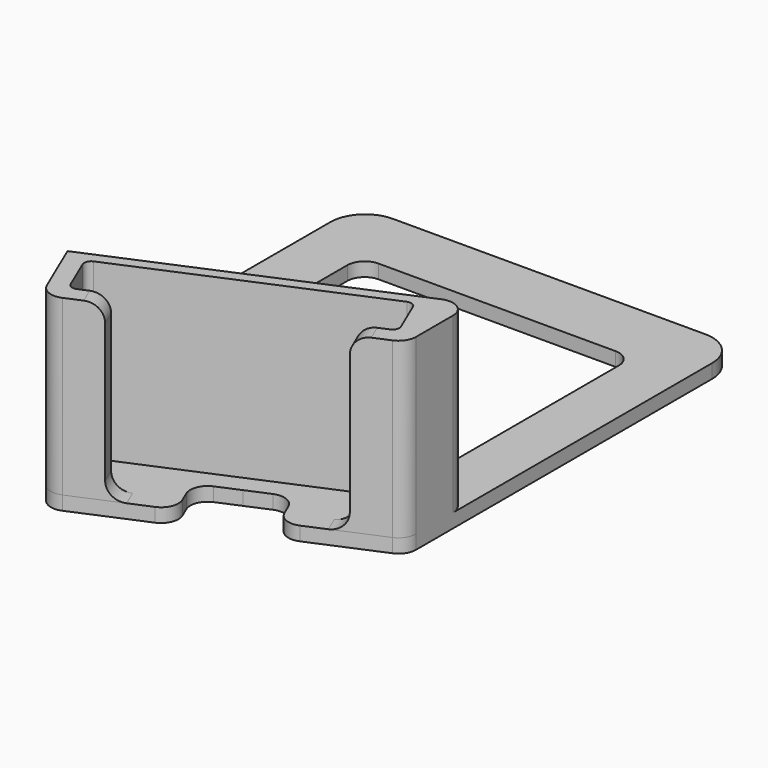
from build123d import *

# Parameters (mm, degrees)
F1_DEPTH  = 4
F2_R      = 5
F4_DEPTH  = 50
F6_DEPTH  = 25
F7_R      = 5
F8_R      = 2
F10_DEPTH = 25
F12_DEPTH = 25
F14_DEPTH = 25
F15_R     = 5


with BuildPart() as f1:
    # F0 (on Top) → F1 (new body)
    with BuildSketch(Plane.XY):
        with BuildLine():
            Line((49.8126317561, 22.0112954478), (-40.1873682439, 22.0112954478))
            ThreePointArc((-40.1873682439, 22.0112954478), (-47.2584360558, 19.0823632597), (-50.1873682439, 12.0112954478))
            Line((-50.1873682439, 12.0112954478), (-50.1873682439, -97.9887045522))
            Line((-50.1873682439, -97.9887045522), (-33.0722484738, -97.9887045522))
            Line((-33.0722484738, -97.9887045522), (59.8126317561, -97.9887045522))
            Line((59.8126317561, -97.9887045522), (59.8126317561, 12.0112954478))
            ThreePointArc((59.8126317561, 12.0112954478), (56.8836995679, 19.0823632597), (49.8126317561, 22.0112954478))
        make_face()
        with BuildLine():
            Line((-34.0809039772, -59.2981277779), (-34.0809039772, -2.0396176167))
            ThreePointArc((-34.0809039772, -2.0396176167), (-32.6164378831, 1.4959162892), (-29.0809039772, 2.9603823833))
            Line((-29.0809039772, 2.9603823833), (39.1555567086, 2.9603823833))
            ThreePointArc((39.1555567086, 2.9603823833), (42.6910906145, 1.4959162892), (44.1555567086, -2.0396176167))
            Line((44.1555567086, -2.0396176167), (44.1555567086, -59.2981277779))
            ThreePointArc((44.1555567086, -59.2981277779), (42.6910906145, -62.8336616838), (39.1555567086, -64.2981277779))
            Line((39.1555567086, -64.2981277779), (-29.0809039772, -64.2981277779))
            ThreePointArc((-29.0809039772, -64.2981277779), (-32.6164378831, -62.8336616838), (-34.0809039772, -59.2981277779))
        make_face(mode=Mode.SUBTRACT)
        Polygon((-18.8066744284, -131.4782482004), (59.8126317561, -97.9887045522), (-33.0722484738, -97.9887045522), align=None)
    extrude(amount=F1_DEPTH)

    # F2
    f2_edges = [f1.edges().sort_by_distance(p)[0] for p in [
        (-33.072248, -97.988705, 2),
        (-50.187368, -97.988705, 2),
        (59.812632, -97.988705, 2),
        (-18.806674, -131.478248, 2),
    ]]
    fillet(f2_edges, radius=F2_R)

    # F3 (on face) → F4 (join)
    with BuildSketch(Plane.XY.offset(4)):
        with BuildLine():
            Line((-6.9660247439, -120.9997456811), (-16.1661150585, -124.9187172558))
            Line((-16.1661150585, -124.9187172558), (-21.6526752631, -112.0385908154))
            Line((-21.6526752631, -112.0385908154), (49.3260715515, -81.8037038021))
            Line((49.3260715515, -81.8037038021), (54.8126317561, -94.6838302426))
            Line((54.8126317561, -94.6838302426), (45.6125414415, -98.6028018173))
            Line((45.6125414415, -98.6028018173), (47.5720272288, -103.2028469746))
            Line((47.5720272288, -103.2028469746), (56.7721175434, -99.2838753999))
            ThreePointArc((56.7721175434, -99.2838753999), (58.9838083848, -97.4408731388), (59.8126317561, -94.6838302426))
            Line((59.8126317561, -94.6838302426), (59.8126317561, -73.8051433371))
            Line((59.8126317561, -73.8051433371), (5.2046610063, -97.0665546714))
            Line((5.2046610063, -97.0665546714), (1.9289534576, -98.4619110571))
            Line((1.9289534576, -98.4619110571), (-23.9415310778, -109.4819869532))
            Line((-23.9415310778, -109.4819869532), (-27.5260314097, -111.0088801064))
            Line((-27.5260314097, -111.0088801064), (-20.7661602158, -126.8782030431))
            ThreePointArc((-20.7661602158, -126.8782030431), (-18.0332724951, -129.5570060682), (-14.2066292711, -129.5187624131))
            Line((-14.2066292711, -129.5187624131), (-5.0065389565, -125.5997908384))
            Line((-5.0065389565, -125.5997908384), (-6.9660247439, -120.9997456811))
        make_face()
        Polygon((-31.7770776261, -101.0292187648), (-27.5260314097, -111.0088801064), (-23.9415310778, -109.4819869532), (-46.2875531446, -57.0229636434), (-49.8720534765, -58.5498567966), align=None)
        Polygon((1.9289534576, -98.4619110571), (5.2046610063, -97.0665546714), (-8.3174404532, -65.3223706937), (-11.5931480018, -66.7177270794), align=None)
    extrude(amount=F4_DEPTH)

    # F5 (on face) → F6 (cut)
    with BuildSketch(Plane.XY.offset(4)):
        Polygon((10.3267065007, -119.0682730989), (21.2827441361, -114.4013189065), (16.1116256489, -102.2617164104), (5.1555880134, -106.9286706028), align=None)
        Polygon((16.1116256489, -102.2617164104), (21.2827441361, -114.4013189065), (32.2387817716, -109.734364714), (27.0676632843, -97.5947622179), align=None)
    extrude(amount=-F6_DEPTH, mode=Mode.SUBTRACT)

    # F7
    f7_edges = [f1.edges().sort_by_distance(p)[0] for p in [
        (-5.986282, -123.299768, 54),
        (46.592284, -100.902824, 54),
        (46.592284, -100.902824, 4),
        (-5.986282, -123.299768, 4),
        (32.238782, -109.734365, 2),
        (10.326707, -119.068273, 2),
        (27.067663, -97.594762, 2),
        (5.155588, -106.928671, 2),
    ]]
    fillet(f7_edges, radius=F7_R)

    # F8
    f8_edges = [f1.edges().sort_by_distance(p)[0] for p in [
        (49.326072, -81.803704, 29),
        (54.812632, -94.68383, 29),
        (-21.652675, -112.038591, 29),
        (-16.166115, -124.918717, 29),
    ]]
    fillet(f8_edges, radius=F8_R)

    # F9 (on face) → F10 (cut)
    with BuildSketch(Plane(origin=(-59.7381223873, -25.4467071035, 0), x_dir=(-0.3918971575, 0.9200090315, 0), z_dir=(0.9200090315, 0.3918971575, 0))):
        Polygon((-34.321681049, 54), (-91.3417988043, 54), (-34.321681049, 4), align=None)
    extrude(amount=-F10_DEPTH, mode=Mode.SUBTRACT)

    # F11 (on face) → F12 (cut)
    with BuildSketch(Plane.XY.offset(4)):
        with BuildLine():
            ThreePointArc((-36.3771227834, -97.9887045522), (-33.6200798872, -98.8175279234), (-31.7770776261, -101.0292187648))
            Line((-31.7770776261, -101.0292187648), (-49.8720534765, -58.5498567966))
            Line((-49.8720534765, -58.5498567966), (-50.1873682439, -57.809630877))
            Line((-50.1873682439, -57.809630877), (-50.1873682439, -92.9887045522))
            ThreePointArc((-50.1873682439, -92.9887045522), (-48.7229021499, -96.5242384581), (-45.1873682439, -97.9887045522))
            Line((-45.1873682439, -97.9887045522), (-36.3771227834, -97.9887045522))
        make_face()
    extrude(amount=-F12_DEPTH, mode=Mode.SUBTRACT)

    # F13 (on face) → F14 (cut)
    with BuildSketch(Plane(origin=(-30.5919303032, -13.0312748216, 0), x_dir=(-0.3918971575, 0.9200090315, 0), z_dir=(0.9200090315, 0.3918971575, 0))):
        Polygon((-56.8375897235, 54), (-91.3417988043, 54), (-56.8375897235, 4), align=None)
    extrude(amount=-F14_DEPTH, mode=Mode.SUBTRACT)

    # F15
    f15_edges = [f1.edges().sort_by_distance(p)[0] for p in [
        (59.812632, -73.805143, 29),
    ]]
    fillet(f15_edges, radius=F15_R)


solid = f1.part
